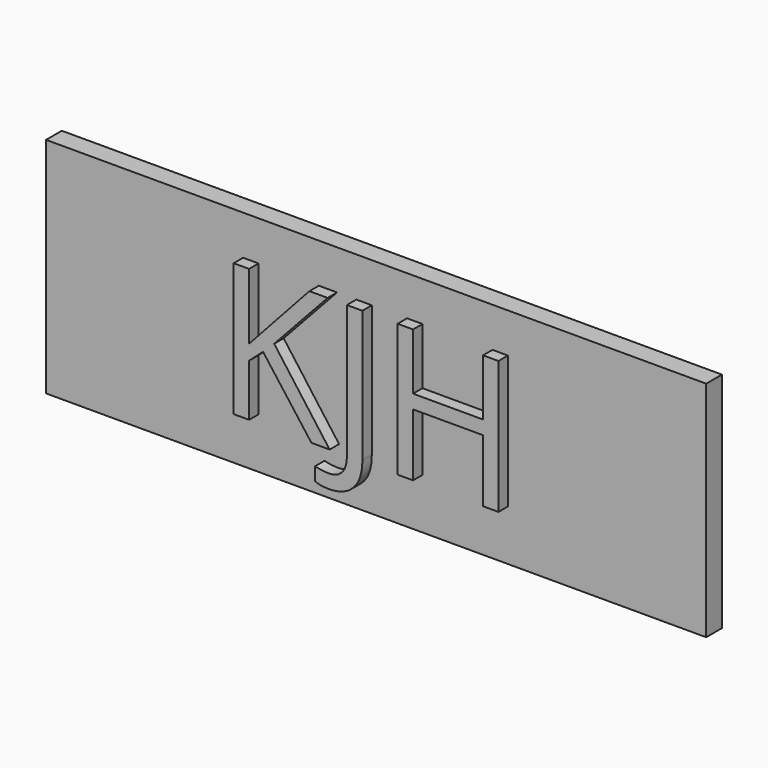
from build123d import *

# Parameters (mm, degrees)
F0_W         = 85.2163881063
F0_H         = 28.82117033
F1_DEPTH     = 2.54
F2_TEXT_SIZE = 24.026012415
F3_DEPTH     = 1.524


# Not quite as in the source:
# - Text() gives the source's letters only with a copy of the font that has no kerning and outlines rounded to 1/6400 em; it was checked with that copy


with BuildPart() as f1:
    # F0 (on Front) → F1 (new body)
    with BuildSketch(Plane.XZ):
        with Locations((42.6081940532, 14.410585165)):
            Rectangle(F0_W, F0_H)
    extrude(amount=F1_DEPTH)

    # F2 (on face) → F3 (join)
    with BuildSketch(Plane.XZ.offset(2.54)):
        with Locations((23.0787522366, 6.5397057298)):
            Text('KJH', F2_TEXT_SIZE, font='Open Sans', text_align=(TextAlign.LEFT, TextAlign.BOTTOM))
    extrude(amount=F3_DEPTH)


solid = f1.part
